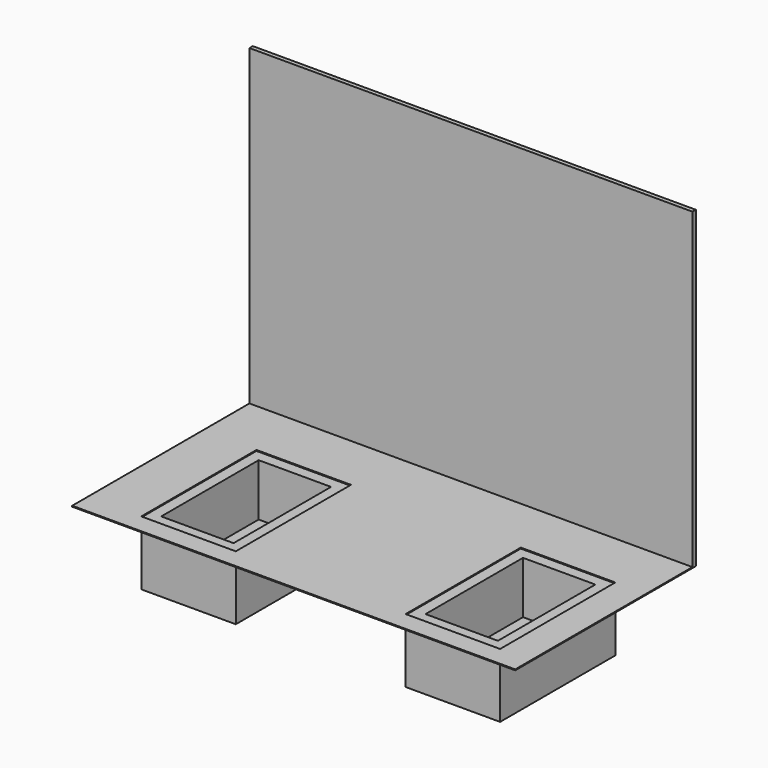
from build123d import *

# Parameters (mm, degrees)
F0_W     = 12000
F0_H     = 114.1832326539
F1_DEPTH = 8500
F0_H_2   = 6000
F0_W_2   = 2560
F0_H_3   = 3900
F2_DEPTH = 25
F0_W_3   = 1960
F0_H_4   = 3300
F3_DEPTH = 1715
F4_T     = -300
F4_2_T   = -300


with BuildPart() as f1:
    # F0 (on Top) → F1 (new body)
    with BuildSketch(Plane.XY):
        with Locations((0, 3062.1825230774)):
            Rectangle(F0_W, F0_H)
    extrude(amount=F1_DEPTH)

    # F0 (on Top) → F2 (join)
    with BuildSketch(Plane.XY):
        with Locations((0, 5.0909067504)):
            Rectangle(F0_W, F0_H_2)
        with Locations((-3273.1487464905, -514.9090932496)):
            Rectangle(F0_W_2, F0_H_3, mode=Mode.SUBTRACT)
        with Locations((3886.8512535095, -514.9090932496)):
            Rectangle(F0_W_2, F0_H_3, mode=Mode.SUBTRACT)
        with Locations((0, 3062.1825230774)):
            Rectangle(F0_W, F0_H)
    extrude(amount=F2_DEPTH)


with BuildPart() as f3:
    # F0 (on Top) → F3 (new body)
    with BuildSketch(Plane.XY):
        with Locations((-3273.1487464905, -514.9090932496)):
            Rectangle(F0_W_2, F0_H_3)
        with Locations((-3273.1487464905, -514.9090932496)):
            Rectangle(F0_W_3, F0_H_4, mode=Mode.SUBTRACT)
        with Locations((-3273.1487464905, -514.9090932496)):
            Rectangle(F0_W_3, F0_H_4)
    extrude(amount=-F3_DEPTH)

    # F4
    f4_openings = [f3.faces().sort_by_distance(p)[0] for p in [
        (-3273.148746, -514.909093, 0),
    ]]
    offset(amount=F4_T, openings=f4_openings)


with BuildPart() as f3b:
    # F0 (on Top) → F3, piece 2 (new body)
    with BuildSketch(Plane.XY):
        with Locations((3886.8512535095, -514.9090932496)):
            Rectangle(F0_W_2, F0_H_3)
        with Locations((3886.8512535095, -514.9090932496)):
            Rectangle(F0_W_3, F0_H_4, mode=Mode.SUBTRACT)
        with Locations((3886.8512535095, -514.9090932496)):
            Rectangle(F0_W_3, F0_H_4)
    extrude(amount=-F3_DEPTH)

    # F4#2
    f4_2_openings = [f3b.faces().sort_by_distance(p)[0] for p in [
        (3886.851254, -514.909093, 0),
    ]]
    offset(amount=F4_2_T, openings=f4_2_openings)


solid = Compound([f1.part, f3.part, f3b.part])
